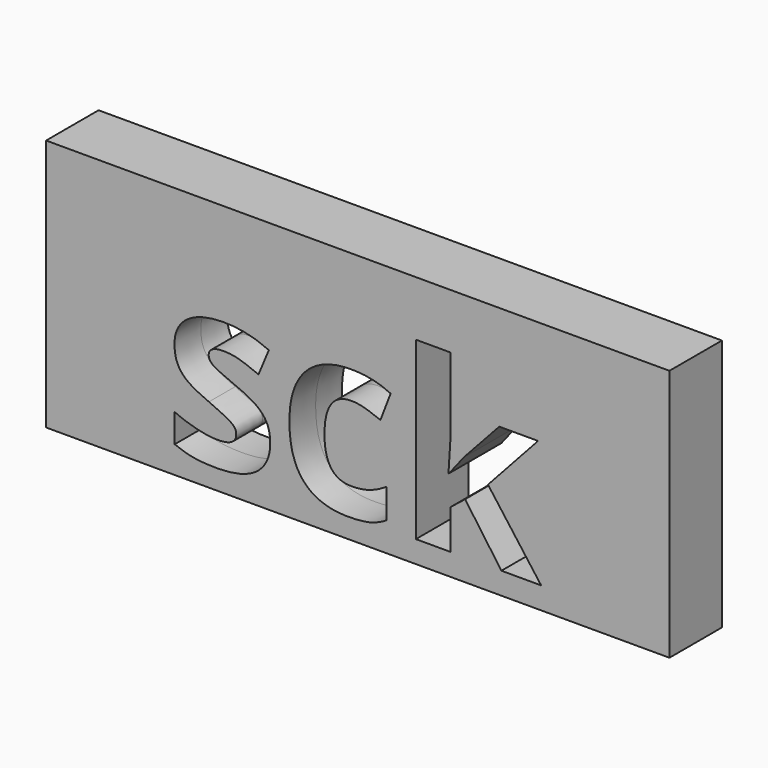
from build123d import *

# Parameters (mm, degrees)
F0_W          = 482.6621413231
F0_H          = 195.6177502871
F1_DEPTH      = 25.4
F1_DEPTH_BACK = 25.4
F2_TEXT_SIZE  = 178.9367550777
F3_DEPTH      = 25.4
F3_DEPTH_BACK = 25.4


# Not quite as in the source:
# - Text() gives the source's letters only with a copy of the font that has no kerning and outlines rounded to 1/6400 em; it was checked with that copy


with BuildPart() as f1:
    # F0 (on Front) → F1 (new body, two sides)
    with BuildSketch(Plane.XZ) as f1_sk:
        with Locations((5.7144165039, 3.6506950855)):
            Rectangle(F0_W, F0_H)
    extrude(amount=F1_DEPTH)
    extrude(f1_sk.sketch, amount=-F1_DEPTH_BACK)

    # F2 (on Front) → F3 (cut, two sides)
    with BuildSketch(Plane.XZ) as f3_sk:
        with Locations((-144.2111423239, -77.1294981241)):
            Text('sck', F2_TEXT_SIZE, font='Open Sans', font_style=FontStyle.BOLD, text_align=(TextAlign.LEFT, TextAlign.BOTTOM))
    extrude(amount=-F3_DEPTH, mode=Mode.SUBTRACT)
    extrude(f3_sk.sketch, amount=F3_DEPTH_BACK, mode=Mode.SUBTRACT)


solid = f1.part
